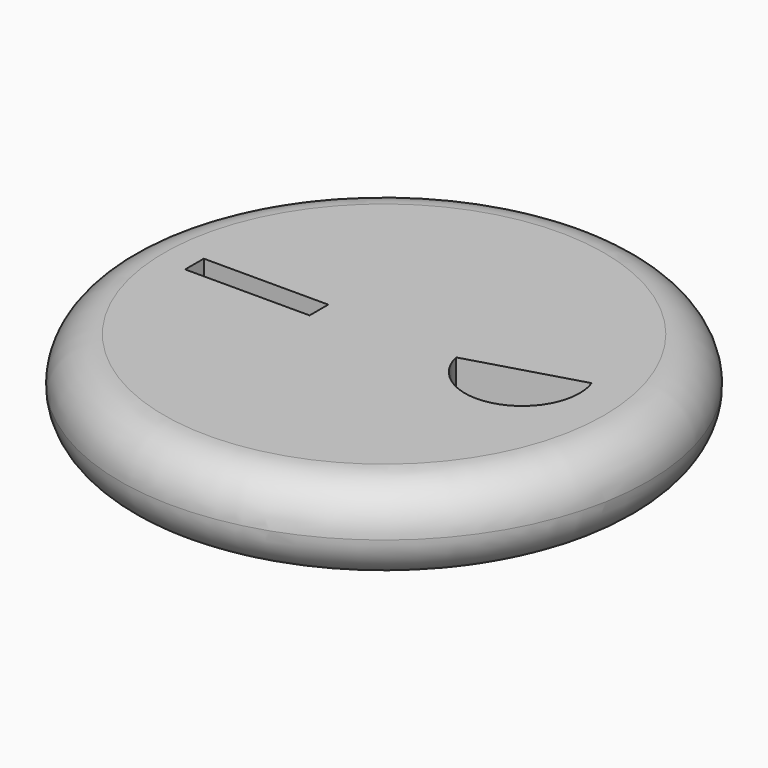
from build123d import *

# Parameters (mm, degrees)
F0_R     = 76.327515992
F0_W     = 35.994451493
F0_H     = 6.7489598878
F1_DEPTH = 25.4
F2_R     = 12.69999


# Not quite as in the source:
# - a fillet or chamfer is up to 0.001 mm smaller than in the source, because OpenCascade refuses the exact size


with BuildPart() as f1:
    # F0 (on Top) → F1 (new body)
    with BuildSketch(Plane.XY):
        Circle(F0_R)
        with BuildLine():
            ThreePointArc((0, 71.7222208521), (50.7152687262, 50.7152687262), (71.7222208521, 0))
            ThreePointArc((71.7222208521, 0), (50.7152687263, -50.7152687262), (0, -71.7222208521))
            ThreePointArc((0, -71.7222208521), (-71.7222208521, 0), (0, 71.7222208521))
        make_face(mode=Mode.SUBTRACT)
        with BuildLine():
            ThreePointArc((0, -71.7222208521), (50.7152687263, -50.7152687262), (71.7222208521, 0))
            ThreePointArc((71.7222208521, 0), (50.7152687262, 50.7152687262), (0, 71.7222208521))
            Line((0, 71.7222208521), (0, -71.7222208521))
        make_face()
        with BuildLine():
            ThreePointArc((51.5885779704, 10.5423588198), (40.6190136024, -10.9400752111), (19.8122242535, 1.2625405457))
            Line((19.8122242535, 1.2625405457), (51.5885779704, 10.5423588198))
        make_face(mode=Mode.SUBTRACT)
        with BuildLine():
            Line((0, -71.7222208521), (0, 71.7222208521))
            ThreePointArc((0, 71.7222208521), (-71.7222208521, 0), (0, -71.7222208521))
        make_face()
        with Locations((-36.8380714208, 0)):
            Rectangle(F0_W, F0_H, mode=Mode.SUBTRACT)
    extrude(amount=F1_DEPTH)

    # F2 (radius 12.7 in the source; OpenCascade refuses exactly that, so slightly less here)
    f2_edges = [f1.edges().sort_by_distance(p)[0] for p in [
        (-76.327516, 0, 25.4),
        (-76.327516, 0, 0),
    ]]
    fillet(f2_edges, radius=F2_R)


solid = f1.part
